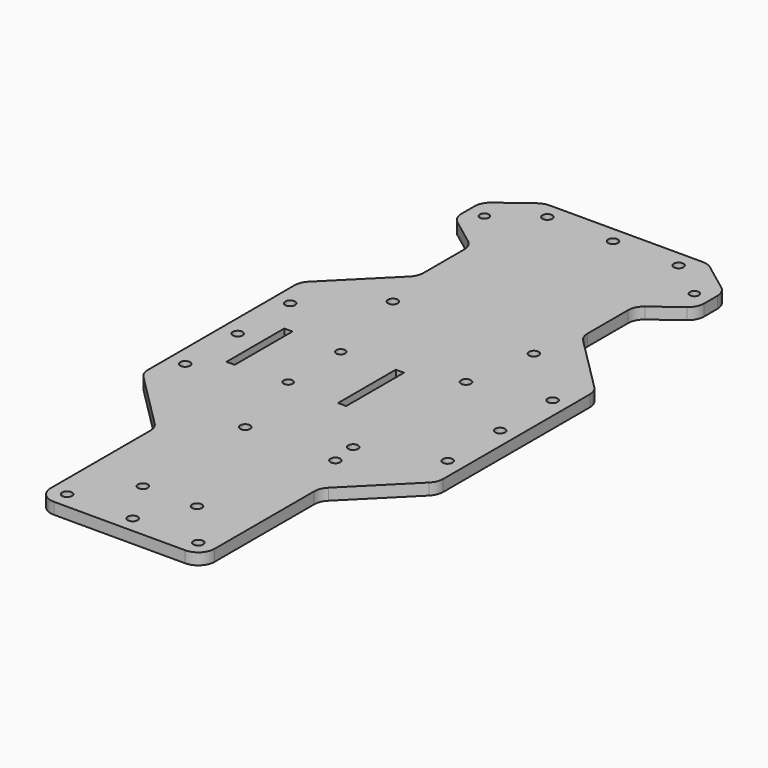
from build123d import *

# Parameters (mm, degrees)
F0_R     = 1.5
F0_W     = 2.5
F0_H     = 22
F0_R_2   = 1.375
F1_DEPTH = 3.5
F2_R     = 5


# Not quite as in the source:
# - a feature names something its author has since deleted; it is built from what else it names


with BuildPart() as f1:
    # F0 (on Top) → F1 (new body)
    with BuildSketch(Plane.XY):
        with BuildLine():
            Line((-25, 52), (-45, 32))
            Line((-45, 32), (-45, -28))
            Line((-45, -28), (-25, -48))
            Line((-25, -48), (-25, -88))
            ThreePointArc((-25, -88), (-23.5355339059, -91.5355339059), (-20, -93))
            Line((-20, -93), (20, -93))
            ThreePointArc((20, -93), (23.5355339059, -91.5355339059), (25, -88))
            Line((25, -88), (25, -48))
            Line((25, -48), (45, -28))
            Line((45, -28), (45, 32))
            Line((45, 32), (25, 52))
            Line((25, 52), (25, 72))
            Line((25, 72), (37, 81))
            Line((37, 81), (37, 91))
            Line((37, 91), (25, 100))
            Line((25, 100), (-25, 100))
            Line((-25, 100), (-37, 91))
            Line((-37, 91), (-37, 81))
            Line((-37, 81), (-25, 72))
            Line((-25, 72), (-25, 52))
        make_face()
        with Locations((-20, -88)):
            Circle(F0_R, mode=Mode.SUBTRACT)
        with Locations((-8.5, -73.5)):
            Circle(F0_R, mode=Mode.SUBTRACT)
        with Locations((-40, -18)):
            Circle(F0_R, mode=Mode.SUBTRACT)
        with Locations((-40, 2)):
            Circle(F0_R, mode=Mode.SUBTRACT)
        with Locations((-31.75, 0)):
            Rectangle(F0_W, F0_H, mode=Mode.SUBTRACT)
        with Locations((-8.5, -34.5)):
            Circle(F0_R, mode=Mode.SUBTRACT)
        with Locations((-15, -10)):
            Circle(F0_R_2, mode=Mode.SUBTRACT)
        with Locations((0, -88)):
            Circle(F0_R, mode=Mode.SUBTRACT)
        with Locations((8, -73.5)):
            Circle(F0_R, mode=Mode.SUBTRACT)
        with Locations((20, -88)):
            Circle(F0_R, mode=Mode.SUBTRACT)
        with Locations((19, -34.5)):
            Circle(F0_R, mode=Mode.SUBTRACT)
        with Locations((18, -26.5)):
            Circle(F0_R, mode=Mode.SUBTRACT)
        with Locations((2.25, 0)):
            Rectangle(F0_W, F0_H, mode=Mode.SUBTRACT)
        with Locations((40, -18)):
            Circle(F0_R, mode=Mode.SUBTRACT)
        with Locations((40, 2)):
            Circle(F0_R, mode=Mode.SUBTRACT)
        with Locations((-40, 22)):
            Circle(F0_R, mode=Mode.SUBTRACT)
        with Locations((-15, 10)):
            Circle(F0_R_2, mode=Mode.SUBTRACT)
        with Locations((-21.5, 38)):
            Circle(F0_R, mode=Mode.SUBTRACT)
        with Locations((-32, 86)):
            Circle(F0_R_2, mode=Mode.SUBTRACT)
        with Locations((-20, 95)):
            Circle(F0_R, mode=Mode.SUBTRACT)
        with Locations((18, 16.5)):
            Circle(F0_R, mode=Mode.SUBTRACT)
        with Locations((21.5, 38)):
            Circle(F0_R, mode=Mode.SUBTRACT)
        with Locations((40, 22)):
            Circle(F0_R, mode=Mode.SUBTRACT)
        with Locations((0, 95)):
            Circle(F0_R, mode=Mode.SUBTRACT)
        with Locations((20, 95)):
            Circle(F0_R, mode=Mode.SUBTRACT)
        with Locations((32, 86)):
            Circle(F0_R_2, mode=Mode.SUBTRACT)
    extrude(amount=F1_DEPTH)

    # F2
    f2_edges = [f1.edges().sort_by_distance(p)[0] for p in [
        (-45, -28, 1.75),
        (-25, -48, 1.75),
        (25, -48, 1.75),
        (45, -28, 1.75),
        (45, 32, 1.75),
        (25, 52, 1.75),
        (25, 72, 1.75),
        (-25, 52, 1.75),
        (-45, 32, 1.75),
        (-25, 72, 1.75),
        (-37, 81, 1.75),
        (-37, 91, 1.75),
        (-25, 100, 1.75),
        (25, 100, 1.75),
        (37, 91, 1.75),
        (37, 81, 1.75),
    ]]
    fillet(f2_edges, radius=F2_R)


solid = f1.part
